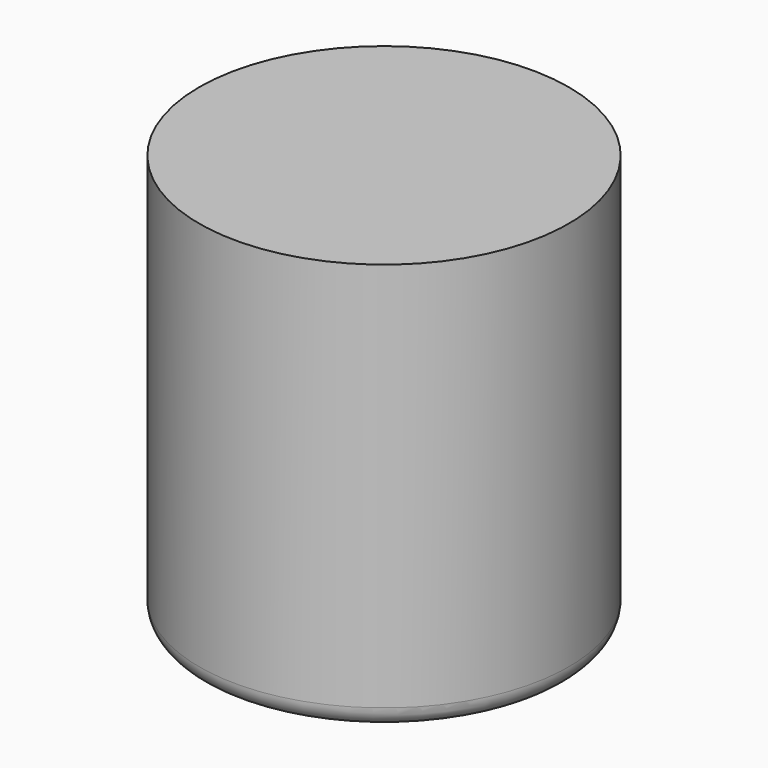
from build123d import *

# Parameters (mm, degrees)
F2_R = 0.5
F3_R = 0.99999


# Not quite as in the source:
# - a fillet or chamfer is up to 0.001 mm smaller than in the source, because OpenCascade refuses the exact size


with BuildPart() as f1:
    # F0 (on Front) → F1 (revolve)
    with BuildSketch(Plane.XZ):
        Polygon((0, 12.7090347865), (0, 14.7090347865), (-9, 14.7090347865), (-9, -5.2909652135), (-7, -5.2909652135), (-7, 12.7090347865), align=None)
    revolve(axis=Axis((0, 0, 4.7090347865), (0, 0, -1)))

    # F2
    f2_edges = [f1.edges().sort_by_distance(p)[0] for p in [
        (7, 0, 12.709035),
    ]]
    fillet(f2_edges, radius=F2_R)

    # F3 (radius 1 in the source; OpenCascade refuses exactly that, so slightly less here)
    f3_edges = [f1.edges().sort_by_distance(p)[0] for p in [
        (9, 0, -5.290965),
        (7, 0, -5.290965),
    ]]
    fillet(f3_edges, radius=F3_R)


solid = f1.part
